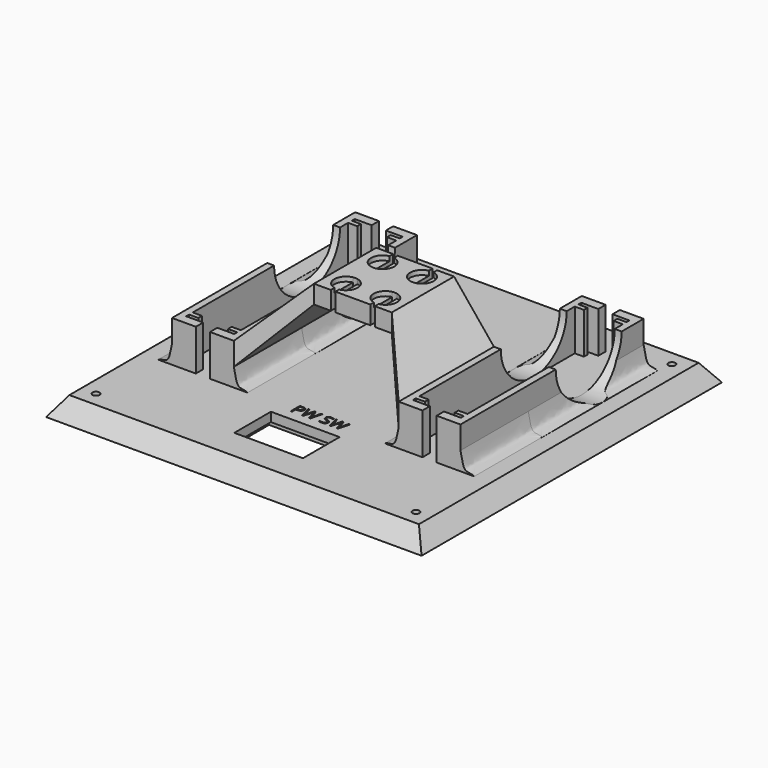
from build123d import *

# Parameters (mm, degrees)
F4_W           = 82
F4_H           = 82
F5_DEPTH       = 4
F5_FACE_W      = 82
F5_FACE_H      = 82
F7_R           = 0.7554422523
F8_DEPTH       = 25
F7_R_2         = 1.5108845046
F9_DEPTH       = 2
F10_W          = 2
F10_H          = 1
F11_DEPTH      = 9
F13_DEPTH      = 18.5
F13_DEPTH_BACK = 31.5
F14_R          = 9
F15_DEPTH      = 50
F15_DEPTH_BACK = 52.3
F16_W          = 15
F16_H          = 10
F17_DEPTH      = 25
F18_W          = 19
F18_H          = 14
F19_DEPTH      = 2
F20_W          = 1
F20_H          = 2
F20_H_2        = 1
F20_W_2        = 2
F20_TEXT_SIZE  = 3.4897976244
F21_DEPTH      = 0.5
F22_DEPTH      = 0.5
F25_DEPTH      = 4
F25_FACE_W     = 17
F25_FACE_H     = 4
F25_FACE1_W    = 17
F25_FACE1_H    = 4
F28_DEPTH      = 3


# Not quite as in the source:
# - Text() gives the source's letters only with a copy of the font that has no kerning and outlines rounded to 1/6400 em; it was checked with that copy


with BuildPart() as f5:
    # F4 (on Top) → F5 (new body)
    with BuildSketch(Plane.XY):
        Rectangle(F4_W, F4_H)
    extrude(amount=F5_DEPTH)

    # F5_face (on face) → F6 section 0
    with BuildSketch(Plane(origin=(0, 0, 0), x_dir=(1, 0, 0), z_dir=(0, 0, -1)), mode=Mode.PRIVATE) as f6_s0:
        Rectangle(F5_FACE_W, F5_FACE_H)
    loft([f6_s0.sketch, Vertex(0, 0, 57.9827560573)], mode=Mode.INTERSECT)

    # F7 (on face) → F8 (cut)
    with BuildSketch(Plane(origin=(0, 0, 0), x_dir=(1, 0, 0), z_dir=(0, 0, -1))):
        with Locations((-34.93934, -34.93934)):
            Circle(F7_R)
        with Locations((-34.93934, 34.93934)):
            Circle(F7_R)
        with Locations((34.93934, 34.93934)):
            Circle(F7_R)
        with Locations((34.93934, -34.93934)):
            Circle(F7_R)
    extrude(amount=-F8_DEPTH, mode=Mode.SUBTRACT)

    # F7 (on face) → F9 (cut)
    with BuildSketch(Plane(origin=(0, 0, 0), x_dir=(1, 0, 0), z_dir=(0, 0, -1))):
        with Locations((-34.93934, 34.93934)):
            Circle(F7_R_2)
        with Locations((-34.93934, 34.93934)):
            Circle(F7_R, mode=Mode.SUBTRACT)
        with Locations((34.93934, 34.93934)):
            Circle(F7_R_2)
        with Locations((34.93934, 34.93934)):
            Circle(F7_R, mode=Mode.SUBTRACT)
        with Locations((-34.93934, -34.93934)):
            Circle(F7_R_2)
        with Locations((-34.93934, -34.93934)):
            Circle(F7_R, mode=Mode.SUBTRACT)
        with Locations((34.93934, -34.93934)):
            Circle(F7_R_2)
        with Locations((34.93934, -34.93934)):
            Circle(F7_R, mode=Mode.SUBTRACT)
    extrude(amount=-F9_DEPTH, mode=Mode.SUBTRACT)

    # F10 (on face) → F11 (join)
    with BuildSketch(Plane.XY.offset(4)):
        Polygon((19.5, 27.7), (19.5, 28.7), (19.5, 29.5), (23.2, 29.5), (23.2, 31.5), (18, 31.5), (18, -18.5), (23.2, -18.5), (23.2, -16.5), (19.5, -16.5), (19.5, -15.7), (19.5, -14.7), align=None)
        Polygon((26.3, -16.5), (26.3, -18.5), (31.5, -18.5), (31.5, 31.5), (26.3, 31.5), (26.3, 29.5), (30, 29.5), (30, 28.7), (30, 27.7), (30, -14.7), (30, -15.7), (30, -16.5), align=None)
        with Locations((20.5, 28.2)):
            Rectangle(F10_W, F10_H)
        with Locations((29, 28.2)):
            Rectangle(F10_W, F10_H)
        with Locations((20.5, -15.2)):
            Rectangle(F10_W, F10_H)
        with Locations((29, -15.2)):
            Rectangle(F10_W, F10_H)
        with Locations((-20.5, -15.2)):
            Rectangle(F10_W, F10_H)
        with Locations((-29, -15.2)):
            Rectangle(F10_W, F10_H)
        Polygon((-30, 28.7), (-30, 29.5), (-26.3, 29.5), (-26.3, 31.5), (-31.5, 31.5), (-31.5, -18.5), (-26.3, -18.5), (-26.3, -16.5), (-30, -16.5), (-30, -15.7), (-30, -14.7), (-30, 27.7), align=None)
        Polygon((-23.2, -16.5), (-23.2, -18.5), (-18, -18.5), (-18, 31.5), (-23.2, 31.5), (-23.2, 29.5), (-19.5, 29.5), (-19.5, 28.7), (-19.5, 27.7), (-19.5, -14.7), (-19.5, -15.7), (-19.5, -16.5), align=None)
        with Locations((-29, 28.2)):
            Rectangle(F10_W, F10_H)
        with Locations((-20.5, 28.2)):
            Rectangle(F10_W, F10_H)
    extrude(amount=F11_DEPTH)

    # F12 (on Front) → F13 (join, two sides)
    with BuildSketch(Plane.XZ) as f13_sk:
        with BuildLine():
            Line((-34.5, 4), (-31.5, 4))
            Line((-31.5, 4), (-31.5, 8))
            add(Edge.make_bspline(
                [(-31.5, 8), (-31.8149834934, 6.9910976287), (-31.9587104101, 3.8985102616), (-33.8204189993, 4.4183517648), (-34.5, 4)],
                knots=[0, 0, 0, 0, 0.5648918788, 1, 1, 1, 1], degree=3))
        make_face()
        with BuildLine():
            add(Edge.make_bspline(
                [(-18, 8), (-17.6850165066, 6.9910976287), (-17.5412895899, 3.8985102616), (-15.6795810007, 4.4183517648), (-15, 4)],
                knots=[0, 0, 0, 0, 0.5648918788, 1, 1, 1, 1], degree=3))
            Line((-18, 8), (-18, 4))
            Line((-18, 4), (-15, 4))
        make_face()
        with BuildLine():
            Line((18, 4), (18, 8))
            add(Edge.make_bspline(
                [(18, 8), (17.6850165066, 6.9910976287), (17.5412895899, 3.8985102616), (15.6795810007, 4.4183517648), (15, 4)],
                knots=[0, 0, 0, 0, 0.5648918788, 1, 1, 1, 1], degree=3))
            Line((15, 4), (18, 4))
        make_face()
        with BuildLine():
            add(Edge.make_bspline(
                [(31.5, 8), (31.8149834934, 6.9910976287), (31.9587104101, 3.8985102616), (33.8204189993, 4.4183517648), (34.5, 4)],
                knots=[0, 0, 0, 0, 0.5648918788, 1, 1, 1, 1], degree=3))
            Line((31.5, 8), (31.5, 4))
            Line((31.5, 4), (34.5, 4))
        make_face()
    extrude(amount=F13_DEPTH)
    extrude(f13_sk.sketch, amount=-F13_DEPTH_BACK)

    # F14 (on Right) → F15 (cut, two sides)
    with BuildSketch(Plane.YZ) as f15_sk:
        with Locations((16.5, 13)):
            Circle(F14_R)
    extrude(amount=-F15_DEPTH, mode=Mode.SUBTRACT)
    extrude(f15_sk.sketch, amount=F15_DEPTH_BACK, mode=Mode.SUBTRACT)

    # F16 (on face) → F17 (cut)
    with BuildSketch(Plane.XY.offset(4)):
        with Locations((0, -26.5)):
            Rectangle(F16_W, F16_H)
    extrude(amount=-F17_DEPTH, mode=Mode.SUBTRACT)

    # F18 (on face) → F19 (cut)
    with BuildSketch(Plane(origin=(0, 0, 0), x_dir=(1, 0, 0), z_dir=(0, 0, -1))):
        with Locations((0, 26.5)):
            Rectangle(F18_W, F18_H)
    extrude(amount=-F19_DEPTH, mode=Mode.SUBTRACT)

    # F20 (on face) → F21 (cut)
    with BuildSketch(Plane.XY.offset(4)):
        with Locations((-24.75, 22.5)):
            Rectangle(F20_W, F20_H)
        with Locations((-24.75, 21)):
            Rectangle(F20_W, F20_H_2)
        with Locations((-26.25, 21)):
            Rectangle(F20_W_2, F20_H_2)
        with Locations((-23.25, 21)):
            Rectangle(F20_W_2, F20_H_2)
        with Locations((-24.75, 19.5)):
            Rectangle(F20_W, F20_H)
        with Locations((24.7, -6.5)):
            Rectangle(F20_W, F20_H)
        with Locations((24.7, -8)):
            Rectangle(F20_W, F20_H_2)
        with Locations((23.2, -8)):
            Rectangle(F20_W_2, F20_H_2)
        with Locations((26.2, -8)):
            Rectangle(F20_W_2, F20_H_2)
        with Locations((24.7, -9.5)):
            Rectangle(F20_W, F20_H)
        with Locations((-5.3202010458, -19.23513785)):
            Text('PW SW', F20_TEXT_SIZE, font='Open Sans', text_align=(TextAlign.LEFT, TextAlign.BOTTOM))
    extrude(amount=-F21_DEPTH, mode=Mode.SUBTRACT)

    # F20 (on face) → F22 (cut)
    with BuildSketch(Plane.XY.offset(4)):
        with Locations((-5.3202010458, -19.23513785)):
            Text('PW SW', F20_TEXT_SIZE, font='Open Sans', text_align=(TextAlign.LEFT, TextAlign.BOTTOM))
    extrude(amount=-F22_DEPTH, mode=Mode.SUBTRACT)



with BuildPart() as f25:
    # F24 (on offset) → F25 (new body)
    with BuildSketch(Plane.XY.offset(19)):
        with BuildLine():
            Line((-4.8, 8.5), (-8.5, 8.5))
            Line((-8.5, 8.5), (-8.5, -8.5))
            Line((-8.5, -8.5), (-4.8, -8.5))
            Line((-4.8, -8.5), (-4.8, -7.50049995))
            ThreePointArc((-4.8, -7.50049995), (-6.85, -5), (-4.8, -2.49950005))
            ThreePointArc((-4.8, -2.49950005), (-4.3, -2.45), (-3.8, -2.49950005))
            ThreePointArc((-3.8, -2.49950005), (-1.75, -5), (-3.8, -7.50049995))
            Line((-3.8, -7.50049995), (-3.8, -8.5))
            Line((-3.8, -8.5), (3.8, -8.5))
            Line((3.8, -8.5), (3.8, -7.50049995))
            ThreePointArc((3.8, -7.50049995), (1.75, -5), (3.8, -2.49950005))
            ThreePointArc((3.8, -2.49950005), (4.3, -2.45), (4.8, -2.49950005))
            ThreePointArc((4.8, -2.49950005), (6.85, -5), (4.8, -7.50049995))
            Line((4.8, -7.50049995), (4.8, -8.5))
            Line((4.8, -8.5), (8.5, -8.5))
            Line((8.5, -8.5), (8.5, 8.5))
            Line((8.5, 8.5), (4.8, 8.5))
            Line((4.8, 8.5), (4.8, 7.50049995))
            ThreePointArc((4.8, 7.50049995), (6.85, 5), (4.8, 2.49950005))
            ThreePointArc((4.8, 2.49950005), (4.3, 2.45), (3.8, 2.49950005))
            ThreePointArc((3.8, 2.49950005), (1.75, 5), (3.8, 7.50049995))
            Line((3.8, 7.50049995), (3.8, 8.5))
            Line((3.8, 8.5), (-3.8, 8.5))
            Line((-3.8, 8.5), (-3.8, 7.50049995))
            ThreePointArc((-3.8, 7.50049995), (-1.75, 5), (-3.8, 2.49950005))
            ThreePointArc((-3.8, 2.49950005), (-4.3, 2.45), (-4.8, 2.49950005))
            ThreePointArc((-4.8, 2.49950005), (-6.85, 5), (-4.8, 7.50049995))
            Line((-4.8, 7.50049995), (-4.8, 8.5))
        make_face()
    extrude(amount=F25_DEPTH)


with BuildPart() as f5_1:
    add(f5.part)

    add(f25.part)  # F26 merges F25
    # F15_face (on face) → F26 section 0
    with BuildSketch(Plane(origin=(-18, -5.2526520745, 10.4766026875), x_dir=(0, 1, 0), z_dir=(1, 0, 0))):
        with BuildLine():
            Line((5.2526520745, -2.4766026875), (14.269337301, -2.4766026875))
            ThreePointArc((14.269337301, -2.4766026875), (13.1401659944, -0.0890887677), (12.7526520745, 2.5233973125))
            Line((12.7526520745, 2.5233973125), (-13.2473479255, 2.5233973125))
            Line((-13.2473479255, 2.5233973125), (-13.2473479255, -2.4766026875))
            Line((-13.2473479255, -2.4766026875), (5.2526520745, -2.4766026875))
        make_face()
    # F25_face (on face) → F26 section 1
    with BuildSketch(Plane(origin=(-8.5, 0, 21), x_dir=(0, -1, 0), z_dir=(-1, 0, 0))):
        Rectangle(F25_FACE_W, F25_FACE_H)
    loft()

    # F15_face1 (on face) → F27 section 0
    with BuildSketch(Plane(origin=(18, -5.2526520745, 10.4766026875), x_dir=(0, -1, 0), z_dir=(-1, 0, 0))):
        with BuildLine():
            Line((-5.2526520745, -2.4766026875), (13.2473479255, -2.4766026875))
            Line((13.2473479255, -2.4766026875), (13.2473479255, 2.5233973125))
            Line((13.2473479255, 2.5233973125), (-12.7526520745, 2.5233973125))
            ThreePointArc((-12.7526520745, 2.5233973125), (-13.1401659944, -0.0890887677), (-14.269337301, -2.4766026875))
            Line((-14.269337301, -2.4766026875), (-5.2526520745, -2.4766026875))
        make_face()
    # F25_face1 (on face) → F27 section 1
    with BuildSketch(Plane(origin=(8.5, 0, 21), x_dir=(0, 1, 0), z_dir=(1, 0, 0))):
        Rectangle(F25_FACE1_W, F25_FACE1_H)
    loft()

    # F24 (on offset) → F28 (join)
    with BuildSketch(Plane.XY.offset(19)):
        with BuildLine():
            Line((-4.8, 8.5), (-8.5, 8.5))
            Line((-8.5, 8.5), (-8.5, -8.5))
            Line((-8.5, -8.5), (-4.8, -8.5))
            Line((-4.8, -8.5), (-4.8, -7.50049995))
            ThreePointArc((-4.8, -7.50049995), (-6.85, -5), (-4.8, -2.49950005))
            ThreePointArc((-4.8, -2.49950005), (-4.3, -2.45), (-3.8, -2.49950005))
            ThreePointArc((-3.8, -2.49950005), (-1.75, -5), (-3.8, -7.50049995))
            Line((-3.8, -7.50049995), (-3.8, -8.5))
            Line((-3.8, -8.5), (3.8, -8.5))
            Line((3.8, -8.5), (3.8, -7.50049995))
            ThreePointArc((3.8, -7.50049995), (1.75, -5), (3.8, -2.49950005))
            ThreePointArc((3.8, -2.49950005), (4.3, -2.45), (4.8, -2.49950005))
            ThreePointArc((4.8, -2.49950005), (6.85, -5), (4.8, -7.50049995))
            Line((4.8, -7.50049995), (4.8, -8.5))
            Line((4.8, -8.5), (8.5, -8.5))
            Line((8.5, -8.5), (8.5, 8.5))
            Line((8.5, 8.5), (4.8, 8.5))
            Line((4.8, 8.5), (4.8, 7.50049995))
            ThreePointArc((4.8, 7.50049995), (6.85, 5), (4.8, 2.49950005))
            ThreePointArc((4.8, 2.49950005), (4.3, 2.45), (3.8, 2.49950005))
            ThreePointArc((3.8, 2.49950005), (1.75, 5), (3.8, 7.50049995))
            Line((3.8, 7.50049995), (3.8, 8.5))
            Line((3.8, 8.5), (-3.8, 8.5))
            Line((-3.8, 8.5), (-3.8, 7.50049995))
            ThreePointArc((-3.8, 7.50049995), (-1.75, 5), (-3.8, 2.49950005))
            ThreePointArc((-3.8, 2.49950005), (-4.3, 2.45), (-4.8, 2.49950005))
            ThreePointArc((-4.8, 2.49950005), (-6.85, 5), (-4.8, 7.50049995))
            Line((-4.8, 7.50049995), (-4.8, 8.5))
        make_face()
        with BuildLine():
            Line((-4.8, 2.49950005), (-4.8, 7.50049995))
            ThreePointArc((-4.8, 7.50049995), (-6.85, 5), (-4.8, 2.49950005))
        make_face()
        with BuildLine():
            ThreePointArc((-4.8, -2.49950005), (-6.85, -5), (-4.8, -7.50049995))
            Line((-4.8, -7.50049995), (-4.8, -2.49950005))
        make_face()
        with BuildLine():
            Line((-3.8, 7.50049995), (-3.8, 2.49950005))
            ThreePointArc((-3.8, 2.49950005), (-1.75, 5), (-3.8, 7.50049995))
        make_face()
        with BuildLine():
            Line((-3.8, -2.49950005), (-3.8, -7.50049995))
            ThreePointArc((-3.8, -7.50049995), (-1.75, -5), (-3.8, -2.49950005))
        make_face()
        with BuildLine():
            ThreePointArc((3.8, -2.49950005), (1.75, -5), (3.8, -7.50049995))
            Line((3.8, -7.50049995), (3.8, -2.49950005))
        make_face()
        with BuildLine():
            Line((4.8, -2.49950005), (4.8, -7.50049995))
            ThreePointArc((4.8, -7.50049995), (6.85, -5), (4.8, -2.49950005))
        make_face()
        with BuildLine():
            Line((3.8, 2.49950005), (3.8, 7.50049995))
            ThreePointArc((3.8, 7.50049995), (1.75, 5), (3.8, 2.49950005))
        make_face()
        with BuildLine():
            ThreePointArc((4.8, 2.49950005), (6.85, 5), (4.8, 7.50049995))
            Line((4.8, 7.50049995), (4.8, 2.49950005))
        make_face()
    extrude(amount=F28_DEPTH)


solid = f5_1.part
